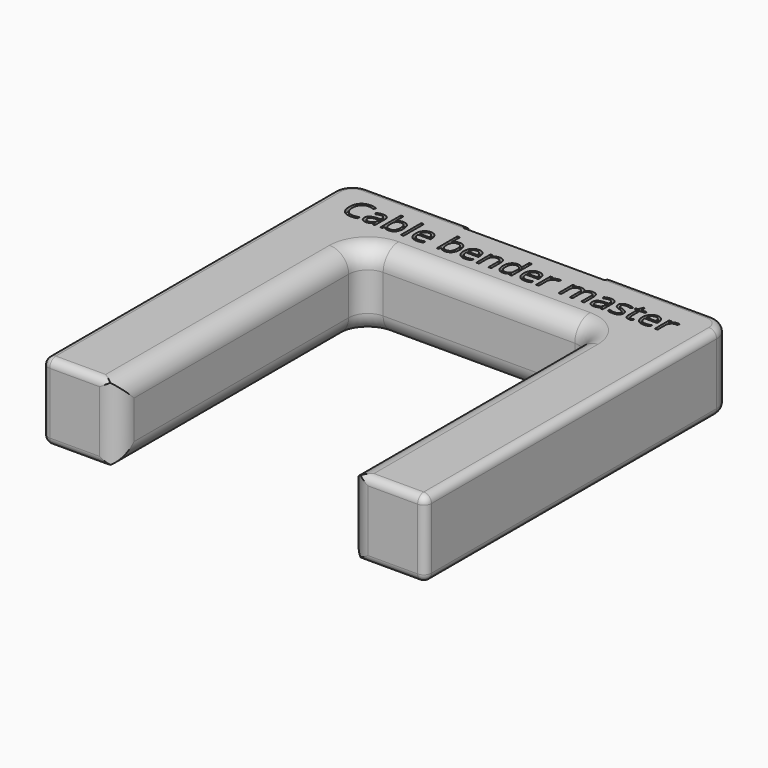
from build123d import *

# Parameters (mm, degrees)
F1_DEPTH      = 10
F1_DEPTH_BACK = 10
F2_R          = 2
F3_DEPTH      = 15
F4_R          = 5
F5_T1_DEPTH   = 93
F5_T3_DEPTH   = 16
F5_T5_DEPTH   = 18
F5_T7_DEPTH   = 18
F5_T9_DEPTH   = 31.5
F5_T11_DEPTH  = 31.5
F5_S15_W      = 2.04
F5_S15_H      = 2.04
F5_T16_DEPTH  = 2.04
F5_S21_W      = 2.04
F5_S21_H      = 2.04
F5_T22_DEPTH  = 2.04
F5_S27_W      = 2.04
F5_S27_H      = 2.04
F5_T28_DEPTH  = 2.04
F5_S33_W      = 2.04
F5_S33_H      = 2.04
F5_T34_DEPTH  = 2.04
F5_T38_ANGLE  = 90
F5_T40_ANGLE  = 90
F5_T42_ANGLE  = 90
F5_T44_ANGLE  = 90
F6_TEXT_SIZE  = 8.7401149681
F7_DEPTH      = 1


# Not quite as in the source:
# - a fillet or chamfer that OpenCascade refuses, or shapes differently, is made with other operations: its cross-section is extruded or revolved along the edge and cut away or added
# - Text() gives the source's letters only with a copy of the font that has no kerning and outlines rounded to 1/6400 em; it was checked with that copy


with BuildPart() as f1:
    # F0 (on Top) → F1 (new body, two sides)
    with BuildSketch(Plane.XY) as f1_sk:
        Polygon((-18.5, 0), (-50, 0), (-50, -100), (-30, -100), (-30, -20), (30, -20), (30, -100), (50, -100), (50, 0), (18.5, 0), (18.5, -2), (-18.5, -2), align=None)
    extrude(amount=F1_DEPTH)
    extrude(f1_sk.sketch, amount=-F1_DEPTH_BACK)

    # F2 (on face) → F3 (cut)
    with BuildSketch(Plane(origin=(0, -2, 0), x_dir=(-1, 0, 0), z_dir=(0, 1, 0))):
        with Locations((-12.5, 5)):
            Circle(F2_R)
        with Locations((12.5, 5)):
            Circle(F2_R)
    extrude(amount=-F3_DEPTH, mode=Mode.SUBTRACT)

    # F4
    f4_edges = [f1.edges().sort_by_distance(p)[0] for p in [
        (50, 0, 0),
        (-50, 0, 0),
        (-30, -100, 0),
        (30, -100, 0),
        (30, -20, 0),
        (-30, -20, 0),
        (0, -20, -10),
        (0, -20, 10),
        (-30, -60, 10),
        (30, -60, 10),
        (-30, -60, -10),
        (30, -60, -10),
    ]]
    fillet(f4_edges, radius=F4_R)

    # F5: fillet of radius 2 on 22 edges, made by hand

    # F5_s2 → F5_t1 (cut)
    with BuildSketch(Plane.XZ.offset(5)):
        with BuildLine():
            ThreePointArc((48, 10), (49.4142135624, 9.4142135624), (50, 8))
            Line((50, 8), (50, 10))
            Line((50, 10), (48, 10))
        make_face()
        with BuildLine():
            ThreePointArc((48, -10), (49.4142135624, -9.4142135624), (50, -8))
            Line((50, -8), (50, -10))
            Line((50, -10), (48, -10))
        make_face()
        with BuildLine():
            ThreePointArc((-48, 10), (-49.4142135624, 9.4142135624), (-50, 8))
            Line((-50, 8), (-50, 10))
            Line((-50, 10), (-48, 10))
        make_face()
        with BuildLine():
            ThreePointArc((-48, -10), (-49.4142135624, -9.4142135624), (-50, -8))
            Line((-50, -8), (-50, -10))
            Line((-50, -10), (-48, -10))
        make_face()
    extrude(amount=F5_T1_DEPTH, mode=Mode.SUBTRACT)

    # F5_s4 → F5_t3 (cut)
    with BuildSketch(Plane.XY.offset(-8)):
        with BuildLine():
            ThreePointArc((50, -98), (49.4142135624, -99.4142135624), (48, -100))
            Line((48, -100), (50, -100))
            Line((50, -100), (50, -98))
        make_face()
        with BuildLine():
            ThreePointArc((-50, -98), (-49.4142135624, -99.4142135624), (-48, -100))
            Line((-48, -100), (-50, -100))
            Line((-50, -100), (-50, -98))
        make_face()
    extrude(amount=F5_T3_DEPTH, mode=Mode.SUBTRACT)

    # F5_s6 → F5_t5 (cut)
    with BuildSketch(Plane.YZ.offset(30)):
        with BuildLine():
            ThreePointArc((-98, 10), (-99.4142135624, 9.4142135624), (-100, 8))
            Line((-100, 8), (-100, 10))
            Line((-100, 10), (-98, 10))
        make_face()
        with BuildLine():
            ThreePointArc((-98, -10), (-99.4142135624, -9.4142135624), (-100, -8))
            Line((-100, -8), (-100, -10))
            Line((-100, -10), (-98, -10))
        make_face()
    extrude(amount=F5_T5_DEPTH, mode=Mode.SUBTRACT)

    # F5_s8 → F5_t7 (cut)
    with BuildSketch(Plane.YZ.offset(-48)):
        with BuildLine():
            ThreePointArc((-98, 10), (-99.4142135624, 9.4142135624), (-100, 8))
            Line((-100, 8), (-100, 10))
            Line((-100, 10), (-98, 10))
        make_face()
        with BuildLine():
            ThreePointArc((-98, -10), (-99.4142135624, -9.4142135624), (-100, -8))
            Line((-100, -8), (-100, -10))
            Line((-100, -10), (-98, -10))
        make_face()
    extrude(amount=F5_T7_DEPTH, mode=Mode.SUBTRACT)

    # F5_s10 → F5_t9 (cut)
    with BuildSketch(Plane.YZ.offset(-45)):
        with BuildLine():
            ThreePointArc((0, 8), (-0.5857864376, 9.4142135624), (-2, 10))
            Line((-2, 10), (0, 10))
            Line((0, 10), (0, 8))
        make_face()
        with BuildLine():
            ThreePointArc((0, -8), (-0.5857864376, -9.4142135624), (-2, -10))
            Line((-2, -10), (0, -10))
            Line((0, -10), (0, -8))
        make_face()
    extrude(amount=F5_T9_DEPTH, mode=Mode.SUBTRACT)

    # F5_s12 → F5_t11 (cut)
    with BuildSketch(Plane.YZ.offset(13.5)):
        with BuildLine():
            ThreePointArc((-2, 10), (-0.5857864376, 9.4142135624), (0, 8))
            Line((0, 8), (0, 10))
            Line((0, 10), (-2, 10))
        make_face()
        with BuildLine():
            ThreePointArc((-2, -10), (-0.5857864376, -9.4142135624), (0, -8))
            Line((0, -8), (0, -10))
            Line((0, -10), (-2, -10))
        make_face()
    extrude(amount=F5_T11_DEPTH, mode=Mode.SUBTRACT)


with BuildPart() as f5_tool14:
    # F5_s15 → F5_t16 (new body)
    with BuildSketch(Plane.XZ.offset(98)):
        with Locations((49.02, 9.02)):
            Rectangle(F5_S15_W, F5_S15_H)
    extrude(amount=F5_T16_DEPTH)

    # F5_s17 → F5_t18 (revolve, cut)
    with BuildSketch(Plane(origin=(48, -98, 8), x_dir=(-0.7071067812, 0, -0.7071067812), z_dir=(-0.7071067812, 0, 0.7071067812))):
        with BuildLine():
            ThreePointArc((0, -2), (2, 0), (0, 2))
            Line((0, 2), (0, -2))
        make_face()
    revolve(axis=Axis((48, -98, 8), (0, -1, 0)), mode=Mode.SUBTRACT)


with BuildPart() as f1_1:
    add(f1.part)

    # F5_t13: cut F5_tool14
    add(f5_tool14.part, mode=Mode.SUBTRACT)


with BuildPart() as f5_tool20:
    # F5_s21 → F5_t22 (new body)
    with BuildSketch(Plane.XZ.offset(98)):
        with Locations((49.02, -9.02)):
            Rectangle(F5_S21_W, F5_S21_H)
    extrude(amount=F5_T22_DEPTH)

    # F5_s23 → F5_t24 (revolve, cut)
    with BuildSketch(Plane(origin=(48, -98, -8), x_dir=(-0.7071067812, 0, 0.7071067812), z_dir=(0.7071067812, 0, 0.7071067812))):
        with BuildLine():
            ThreePointArc((0, -2), (2, 0), (0, 2))
            Line((0, 2), (0, -2))
        make_face()
    revolve(axis=Axis((48, -98, -8), (0, -1, 0)), mode=Mode.SUBTRACT)


with BuildPart() as f1_2:
    add(f1_1.part)

    # F5_t19: cut F5_tool20
    add(f5_tool20.part, mode=Mode.SUBTRACT)


with BuildPart() as f5_tool26:
    # F5_s27 → F5_t28 (new body)
    with BuildSketch(Plane.XY.offset(8)):
        with Locations((-49.02, -99.02)):
            Rectangle(F5_S27_W, F5_S27_H)
    extrude(amount=F5_T28_DEPTH)

    # F5_s29 → F5_t30 (revolve, cut)
    with BuildSketch(Plane(origin=(-48, -98, 8), x_dir=(0.7071067812, 0.7071067812, 0), z_dir=(0.7071067812, -0.7071067812, 0))):
        with BuildLine():
            ThreePointArc((0, -2), (2, 0), (0, 2))
            Line((0, 2), (0, -2))
        make_face()
    revolve(axis=Axis((-48, -98, 8), (0, 0, 1)), mode=Mode.SUBTRACT)


with BuildPart() as f1_3:
    add(f1_2.part)

    # F5_t25: cut F5_tool26
    add(f5_tool26.part, mode=Mode.SUBTRACT)


with BuildPart() as f5_tool32:
    # F5_s33 → F5_t34 (new body)
    with BuildSketch(Plane.XY.offset(-8)):
        with Locations((-49.02, -99.02)):
            Rectangle(F5_S33_W, F5_S33_H)
    extrude(amount=-F5_T34_DEPTH)

    # F5_s35 → F5_t36 (revolve, cut)
    with BuildSketch(Plane(origin=(-48, -98, -8), x_dir=(0.7071067812, 0.7071067812, 0), z_dir=(-0.7071067812, 0.7071067812, 0))):
        with BuildLine():
            ThreePointArc((0, -2), (2, 0), (0, 2))
            Line((0, 2), (0, -2))
        make_face()
    revolve(axis=Axis((-48, -98, -8), (0, 0, -1)), mode=Mode.SUBTRACT)


with BuildPart() as f1_4:
    add(f1_3.part)

    # F5_t31: cut F5_tool32
    add(f5_tool32.part, mode=Mode.SUBTRACT)

    # F5_s37 → F5_t38 (revolve, cut)
    with BuildSketch(Plane.YZ.offset(-45)):
        with BuildLine():
            ThreePointArc((-2, 10), (-0.5857864376, 9.4142135624), (0, 8))
            Line((0, 8), (0, 10))
            Line((0, 10), (-2, 10))
        make_face()
    revolve(axis=Axis((-45, -5, 10), (0, 0, 1)), revolution_arc=F5_T38_ANGLE, mode=Mode.SUBTRACT)

    # F5_s39 → F5_t40 (revolve, cut)
    with BuildSketch(Plane.XZ.offset(5)):
        with BuildLine():
            ThreePointArc((48, 10), (49.4142135624, 9.4142135624), (50, 8))
            Line((50, 8), (50, 10))
            Line((50, 10), (48, 10))
        make_face()
    revolve(axis=Axis((45, -5, 10), (0, 0, 1)), revolution_arc=F5_T40_ANGLE, mode=Mode.SUBTRACT)

    # F5_s41 → F5_t42 (revolve, cut)
    with BuildSketch(Plane.YZ.offset(-45)):
        with BuildLine():
            ThreePointArc((0, -8), (-0.5857864376, -9.4142135624), (-2, -10))
            Line((-2, -10), (0, -10))
            Line((0, -10), (0, -8))
        make_face()
    revolve(axis=Axis((-45, -5, -10), (0, 0, 1)), revolution_arc=F5_T42_ANGLE, mode=Mode.SUBTRACT)

    # F5_s43 → F5_t44 (revolve, cut)
    with BuildSketch(Plane.XZ.offset(5)):
        with BuildLine():
            ThreePointArc((48, -10), (49.4142135624, -9.4142135624), (50, -8))
            Line((50, -8), (50, -10))
            Line((50, -10), (48, -10))
        make_face()
    revolve(axis=Axis((45, -5, -10), (0, 0, 1)), revolution_arc=F5_T44_ANGLE, mode=Mode.SUBTRACT)

    # F6 (on face) → F7 (cut)
    with BuildSketch(Plane.XY.offset(10)):
        with Locations((-43, -12.3040768929)):
            Text('Cable bender master', F6_TEXT_SIZE, font='Open Sans', text_align=(TextAlign.LEFT, TextAlign.BOTTOM))
    extrude(amount=-F7_DEPTH, mode=Mode.SUBTRACT)


solid = f1_4.part
